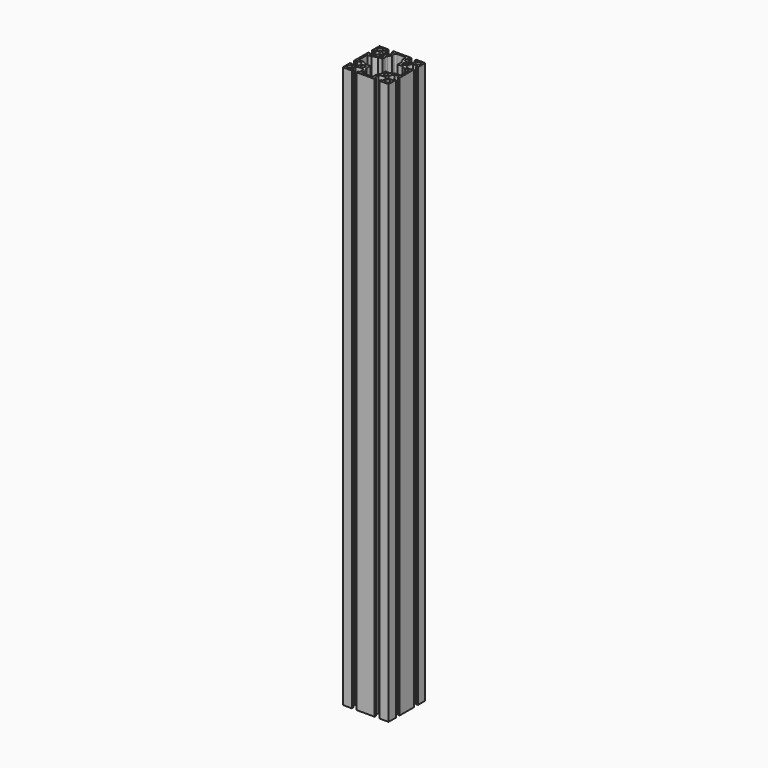
from build123d import *

# Parameters (mm, degrees)
F0_R     = 3
F0_R_2   = 2.5
F1_DEPTH = 735
F2_R     = 2
F3_R     = 7


# Not quite as in the source:
# - a feature names something its author has since deleted; it is built from what else it names


with BuildPart() as f1:
    # F0 (on Top) → F1 (new body)
    with BuildSketch(Plane.XY):
        with BuildLine():
            Line((18.15, -30), (30, -30))
            Line((30, -30), (30, -18.15))
            Line((30, -18.15), (27.5, -18.15))
            Line((27.5, -18.15), (27.5, -20.15))
            Line((27.5, -20.15), (21.5477069044, -20.15))
            ThreePointArc((21.5477069044, -20.15), (19.5, -15), (21.5477069044, -9.85))
            Line((21.5477069044, -9.85), (27.5, -9.85))
            Line((27.5, -9.85), (27.5, -11.85))
            Line((27.5, -11.85), (30, -11.85))
            Line((30, -11.85), (30, 11.85))
            Line((30, 11.85), (27.5, 11.85))
            Line((27.5, 11.85), (27.5, 9.85))
            Line((27.5, 9.85), (21.5477069044, 9.85))
            ThreePointArc((21.5477069044, 9.85), (19.5, 15), (21.5477069044, 20.15))
            Line((21.5477069044, 20.15), (27.5, 20.15))
            Line((27.5, 20.15), (27.5, 18.15))
            Line((27.5, 18.15), (30, 18.15))
            Line((30, 18.15), (30, 30))
            Line((30, 30), (18.15, 30))
            Line((18.15, 30), (18.15, 27.5))
            Line((18.15, 27.5), (20.15, 27.5))
            Line((20.15, 27.5), (20.15, 21.5477069044))
            ThreePointArc((20.15, 21.5477069044), (15, 19.5), (9.85, 21.5477069044))
            Line((9.85, 21.5477069044), (9.85, 27.5))
            Line((9.85, 27.5), (11.85, 27.5))
            Line((11.85, 27.5), (11.85, 30))
            Line((11.85, 30), (-11.85, 30))
            Line((-11.85, 30), (-11.85, 27.5))
            Line((-11.85, 27.5), (-9.85, 27.5))
            Line((-9.85, 27.5), (-9.85, 21.5477069044))
            ThreePointArc((-9.85, 21.5477069044), (-15, 19.5), (-20.15, 21.5477069044))
            Line((-20.15, 21.5477069044), (-20.15, 27.5))
            Line((-20.15, 27.5), (-18.15, 27.5))
            Line((-18.15, 27.5), (-18.15, 30))
            Line((-18.15, 30), (-30, 30))
            Line((-30, 30), (-30, 18.15))
            Line((-30, 18.15), (-27.5, 18.15))
            Line((-27.5, 18.15), (-27.5, 20.15))
            Line((-27.5, 20.15), (-21.5477069044, 20.15))
            ThreePointArc((-21.5477069044, 20.15), (-19.5, 15), (-21.5477069044, 9.85))
            Line((-21.5477069044, 9.85), (-27.5, 9.85))
            Line((-27.5, 9.85), (-27.5, 11.85))
            Line((-27.5, 11.85), (-30, 11.85))
            Line((-30, 11.85), (-30, -11.85))
            Line((-30, -11.85), (-27.5, -11.85))
            Line((-27.5, -11.85), (-27.5, -9.85))
            Line((-27.5, -9.85), (-21.5477069044, -9.85))
            ThreePointArc((-21.5477069044, -9.85), (-19.5, -15), (-21.5477069044, -20.15))
            Line((-21.5477069044, -20.15), (-27.5, -20.15))
            Line((-27.5, -20.15), (-27.5, -18.15))
            Line((-27.5, -18.15), (-30, -18.15))
            Line((-30, -18.15), (-30, -30))
            Line((-30, -30), (-18.15, -30))
            Line((-18.15, -30), (-18.15, -27.5))
            Line((-18.15, -27.5), (-20.15, -27.5))
            Line((-20.15, -27.5), (-20.15, -21.5477069044))
            ThreePointArc((-20.15, -21.5477069044), (-15, -19.5), (-9.85, -21.5477069044))
            Line((-9.85, -21.5477069044), (-9.85, -27.5))
            Line((-9.85, -27.5), (-11.85, -27.5))
            Line((-11.85, -27.5), (-11.85, -30))
            Line((-11.85, -30), (11.85, -30))
            Line((11.85, -30), (11.85, -27.5))
            Line((11.85, -27.5), (9.85, -27.5))
            Line((9.85, -27.5), (9.85, -21.5477069044))
            ThreePointArc((9.85, -21.5477069044), (15, -19.5), (20.15, -21.5477069044))
            Line((20.15, -21.5477069044), (20.15, -27.5))
            Line((20.15, -27.5), (18.15, -27.5))
            Line((18.15, -27.5), (18.15, -30))
        make_face()
        with Locations((-25, -25)):
            Circle(F0_R, mode=Mode.SUBTRACT)
        with Locations((-15, -15)):
            Circle(F0_R_2, mode=Mode.SUBTRACT)
        with Locations((25, -25)):
            Circle(F0_R, mode=Mode.SUBTRACT)
        with Locations((15, -15)):
            Circle(F0_R_2, mode=Mode.SUBTRACT)
        with Locations((-25, 25)):
            Circle(F0_R, mode=Mode.SUBTRACT)
        with Locations((-15, 15)):
            Circle(F0_R_2, mode=Mode.SUBTRACT)
        Polygon((-7, 22), (-7, 27.5), (0, 27.5), (7, 27.5), (7, 22), (10, 16), (10, 10), (16, 10), (22, 7), (27.5, 7), (27.5, 0), (27.5, -7), (22, -7), (16, -10), (10, -10), (10, -16), (7, -22), (7, -27.5), (0, -27.5), (-7, -27.5), (-7, -22), (-10, -16), (-10, -10), (-16, -10), (-22, -7), (-27.5, -7), (-27.5, 0), (-27.5, 7), (-22, 7), (-16, 10), (-10, 10), (-10, 16), align=None, mode=Mode.SUBTRACT)
        with Locations((15, 15)):
            Circle(F0_R_2, mode=Mode.SUBTRACT)
        with Locations((25, 25)):
            Circle(F0_R, mode=Mode.SUBTRACT)
    extrude(amount=F1_DEPTH)

    # F2
    f2_edges = [f1.edges().sort_by_distance(p)[0] for p in [
        (-7, 27.5, 367.5),
        (7, 27.5, 367.5),
    ]]
    fillet(f2_edges, radius=F2_R)

    # F3
    f3_edges = [f1.edges().sort_by_distance(p)[0] for p in [
        (-10, 16, 367.5),
        (10, 16, 367.5),
    ]]
    fillet(f3_edges, radius=F3_R)


solid = f1.part
